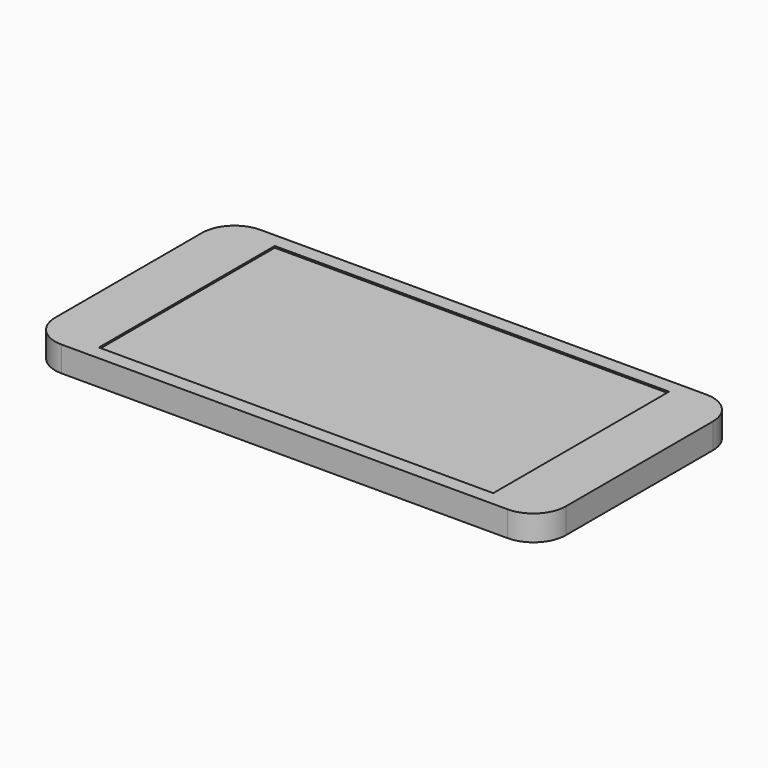
from build123d import *

# Parameters (mm, degrees)
F0_W     = 158
F0_H     = 7.87
F1_DEPTH = 38.435
F2_R     = 10
F3_W     = 122
F3_H     = 68
F4_DEPTH = 0.5
F7_R     = 3.5
F8_DEPTH = 1


# Not quite as in the source:
# - the program builds the solid bodies; features that only make, move or delete a surface that nothing else refers to are left out


with BuildPart() as f1:
    # F0 (on Front) → F1 (new body, symmetric)
    with BuildSketch(Plane.XZ):
        Rectangle(F0_W, F0_H)
    extrude(amount=F1_DEPTH, both=True)

    # F2
    f2_edges = [f1.edges().sort_by_distance(p)[0] for p in [
        (-79, 38.435, 0),
        (-79, -38.435, 0),
        (79, -38.435, 0),
        (79, 38.435, 0),
    ]]
    fillet(f2_edges, radius=F2_R)

    # F3 (on face) → F4 (cut)
    with BuildSketch(Plane.XY.offset(3.935)):
        Rectangle(F3_W, F3_H)
    extrude(amount=-F4_DEPTH, mode=Mode.SUBTRACT)

    # F7 (on face) → F8 (cut)
    with BuildSketch(Plane(origin=(0, 0, -3.935), x_dir=(1, 0, 0), z_dir=(0, 0, -1))):
        with Locations((-72, -24.435)):
            Circle(F7_R)
    extrude(amount=-F8_DEPTH, mode=Mode.SUBTRACT)


solid = f1.part
